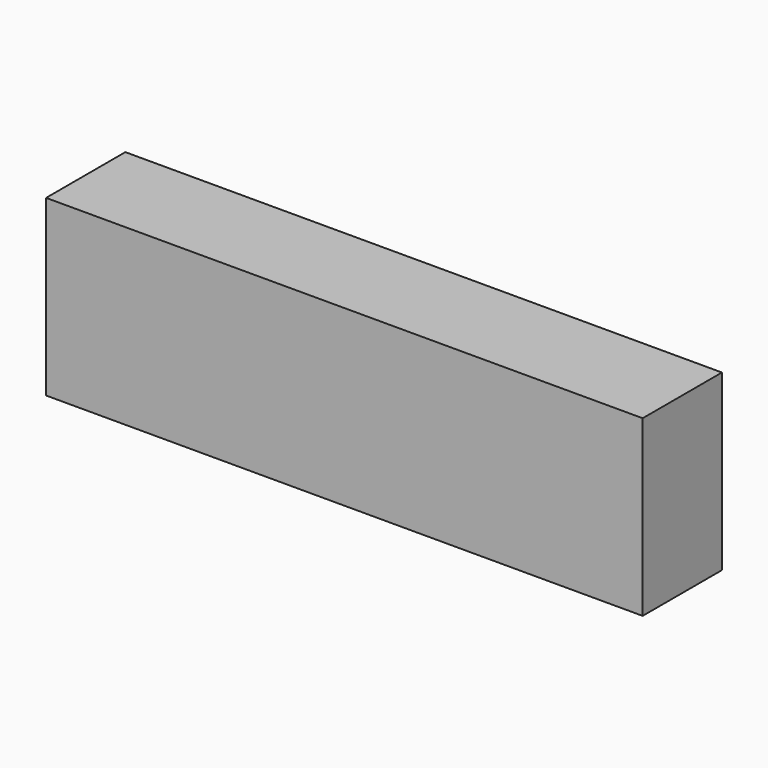
from build123d import *

# Parameters (mm, degrees)
F0_W     = 87.0870612562
F0_H     = 14.461196959
F1_DEPTH = 25.4


# Not quite as in the source:
# - a feature names something its author has since deleted; it is built from what else it names


with BuildPart() as f1:
    # F0 (on Top) → F1 (new body)
    with BuildSketch(Plane.XY):
        with Locations((13.4609509259, -39.1359739006)):
            Rectangle(F0_W, F0_H)
    extrude(amount=F1_DEPTH)


solid = f1.part
